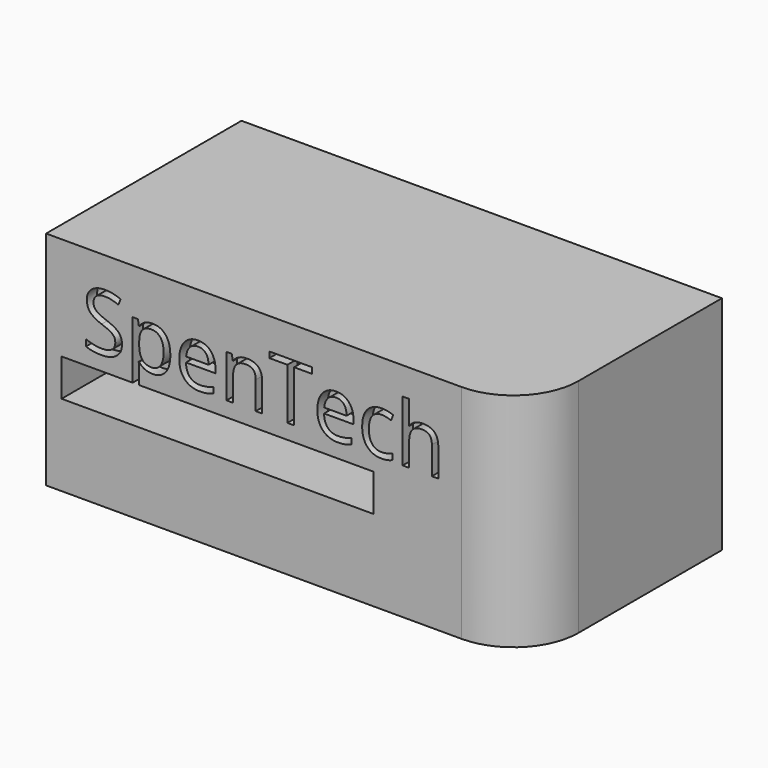
from build123d import *

# Parameters (mm, degrees)
F0_W         = 130.423642695
F0_H         = 60.1940229535
F2_DEPTH     = 66.3
F3_W         = 84.671664983
F3_H         = 10.1100495085
F5_DEPTH     = 31.1
F6_TEXT_SIZE = 21.6909283255
F7_DEPTH     = 3.5
F8_R         = 17.6237590053


# Not quite as in the source:
# - Text() gives the source's letters only with a copy of the font that has no kerning and outlines rounded to 1/6400 em; it was checked with that copy


with BuildPart() as f2:
    # F0 (on Front) → F2 (new body)
    with BuildSketch(Plane.XZ):
        with Locations((-6.8440176547, 2.9402971268)):
            Rectangle(F0_W, F0_H)
    extrude(amount=F2_DEPTH)

    # F3 (on face) → F5 (cut)
    with BuildSketch(Plane.XZ.offset(66.3)):
        with Locations((-25.5123805255, -0.0283638947)):
            Rectangle(F3_W, F3_H)
    extrude(amount=-F5_DEPTH, mode=Mode.SUBTRACT)

    # F6 (on face) → F7 (cut)
    with BuildSketch(Plane.XZ.offset(66.3)):
        with Locations((-62.319047749, 9.0861404315)):
            Text('SpenTech', F6_TEXT_SIZE, font='Open Sans', text_align=(TextAlign.LEFT, TextAlign.BOTTOM))
    extrude(amount=-F7_DEPTH, mode=Mode.SUBTRACT)

    # F8
    f8_edges = [f2.edges().sort_by_distance(p)[0] for p in [
        (58.367804, -66.3, 2.940297),
    ]]
    fillet(f8_edges, radius=F8_R)


solid = f2.part
